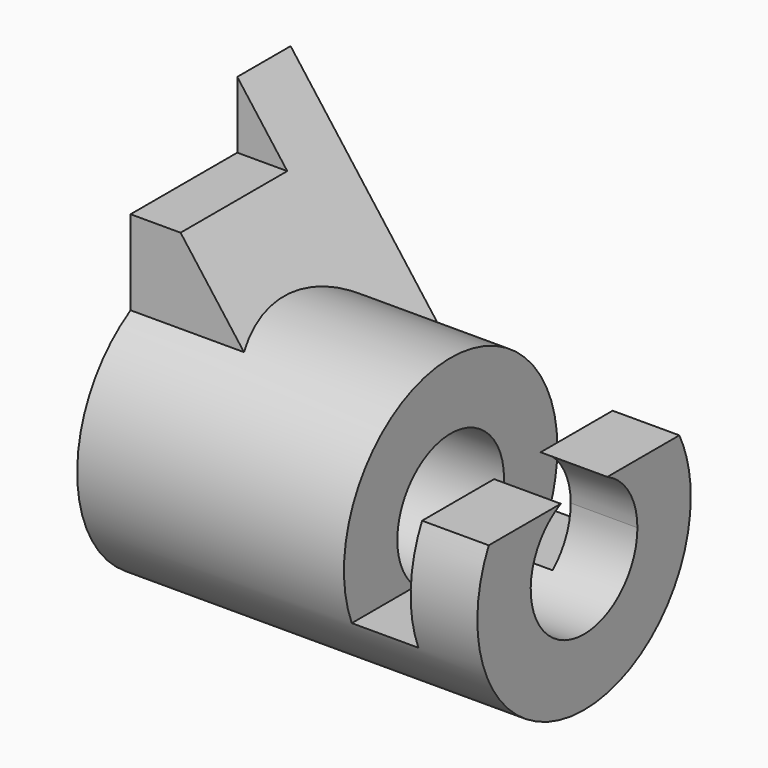
from build123d import *
from build123d import SkipClean  # not in build123d's __all__

# Parameters (mm, degrees)
F0_R           = 25.4
F0_R_2         = 12.7
F1_DEPTH       = 50.8
F3_DEPTH       = 38.1
F5_DEPTH       = 50.801
F6_DEPTH       = 25.4
F7_DEPTH       = 50.801
F9_DEPTH       = 25.4
F10_W          = 12.7
F10_H          = 34.925
F11_DEPTH      = 25.401
F11_DEPTH_BACK = 25.4


# Not quite as in the source:
# - a feature names something its author has since deleted; it is built from what else it names


with BuildPart() as f1:
    # F0 (on Right) → F1 (new body)
    with BuildSketch(Plane.YZ):
        Circle(F0_R)
        Circle(F0_R_2, mode=Mode.SUBTRACT)
    extrude(amount=F1_DEPTH)

    # F2 (on Right) → F3 (join)
    with BuildSketch(Plane.YZ):
        Polygon((-12.7, 38.1), (-12.7, 0), (25.4, 0), (25.4, 50.8), (12.7, 50.8), (12.7, 38.1), align=None)
    extrude(amount=F3_DEPTH)

    # F4 (on face) → F5 (cut, through all)
    with BuildSketch(Plane(origin=(0, 25.4, 0), x_dir=(-1, 0, 0), z_dir=(0, 1, 0))):
        Polygon((-38.1, 0), (0, 50.8), (-38.1, 50.8), align=None)
    extrude(amount=-F5_DEPTH, mode=Mode.SUBTRACT)

    # F6 (add): a face of the model
    f6_faces = [f1.faces().sort_by_distance(p)[0] for p in [
        (38.1, 19.05, 0.5679612663),
    ]]
    extrude(f6_faces, amount=F6_DEPTH)

    # F0 (on Right) → F7 (cut, through all)
    with BuildSketch(Plane.YZ):
        Circle(F0_R_2)
    extrude(amount=F7_DEPTH, mode=Mode.SUBTRACT)

    # F8 (on face) → F9 (join)
    with BuildSketch(Plane.YZ.offset(50.8)):
        with BuildLine():
            Line((-5.5358016583, 11.43), (-22.6829252964, 11.43))
            ThreePointArc((-22.6829252964, 11.43), (-5.8742530365, -24.7113971937), (25.4, 0))
            ThreePointArc((25.4, 0), (24.7113971937, 5.8742530365), (22.6829252964, 11.43))
            Line((22.6829252964, 11.43), (5.5358016583, 11.43))
            ThreePointArc((5.5358016583, 11.43), (10.7609172718, 6.7448246434), (12.7, 0))
            ThreePointArc((12.7, 0), (-6.7448246434, -10.7609172718), (-5.5358016583, 11.43))
        make_face()
    with SkipClean():  # cleaning this boolean's faces spoils the solid; the shape is the same uncleaned
        extrude(amount=F9_DEPTH)

    # F10 (on Front) → F11 (cut, two sides)
    with BuildSketch(Plane.XZ) as f11_sk:
        with Locations((57.15, 7.9375)):
            Rectangle(F10_W, F10_H)
    extrude(amount=-F11_DEPTH, mode=Mode.SUBTRACT)
    extrude(f11_sk.sketch, amount=F11_DEPTH_BACK, mode=Mode.SUBTRACT)


solid = f1.part
